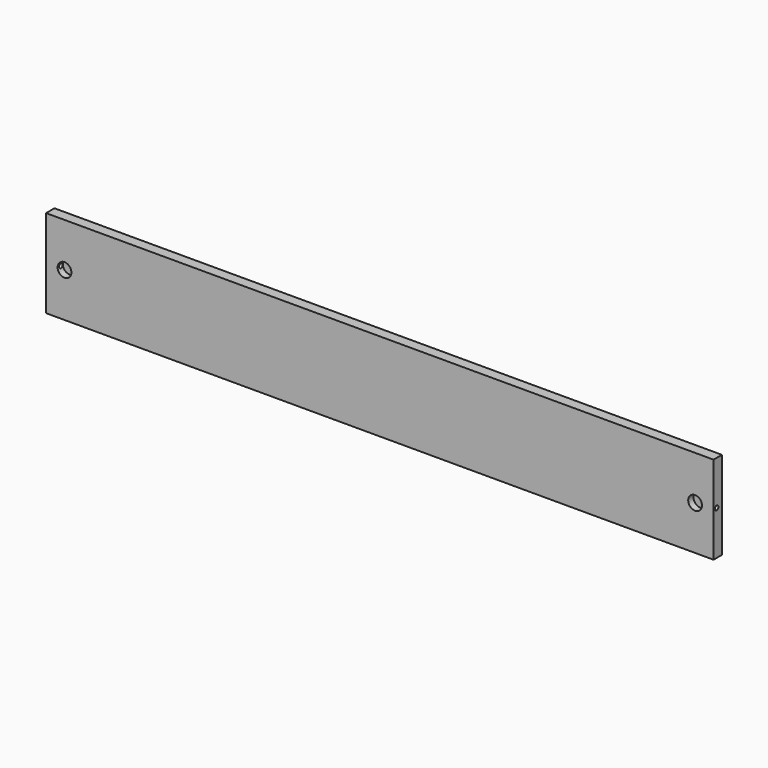
from build123d import *

# Parameters (mm, degrees)
F0_W     = 1212
F0_H     = 160
F1_DEPTH = 19
F2_R     = 12.5
F3_DEPTH = 12
F5_D     = 8
F5_DEPTH = 22
F5_TIP   = 2.4034424761


# Not quite as in the source:
# - a pattern or mirror of a feature is missing from the dataset's text; its kind, count and spacing are read off the source's solid


with BuildPart() as f1:
    # F0 (on Front) → F1 (new body)
    with BuildSketch(Plane.XZ):
        Rectangle(F0_W, F0_H)
    extrude(amount=F1_DEPTH)

    # F2 (on face) → F3 (cut)
    with BuildSketch(Plane.XZ.offset(19)):
        with Locations((-572.5, 0)):
            Circle(F2_R)
    f3 = extrude(amount=-F3_DEPTH, mode=Mode.SUBTRACT)

    # F3_copies: F3 across plane
    add(f3.mirror(Plane(origin=(0, 0, 0), x_dir=(0, 0, 1), z_dir=(1, 0, 0))), mode=Mode.SUBTRACT)

    # F5
    with Locations(Plane(origin=(-606, 0, 0), x_dir=(0, -1, 0), z_dir=(-1, 0, 0))):
        with Locations((12, 0)):
            f5 = Hole(F5_D / 2, depth=F5_DEPTH)
            with Locations((0, 0, -(F5_DEPTH + F5_TIP / 2))):  # 118° drill point
                Cone(0, F5_D / 2, F5_TIP, mode=Mode.SUBTRACT)

    # F5_copies: F5 across plane
    add(f5.mirror(Plane(origin=(3.5e-05, 0, 0), x_dir=(0, 0, 1), z_dir=(1, 0, 0))), mode=Mode.SUBTRACT)


solid = f1.part
